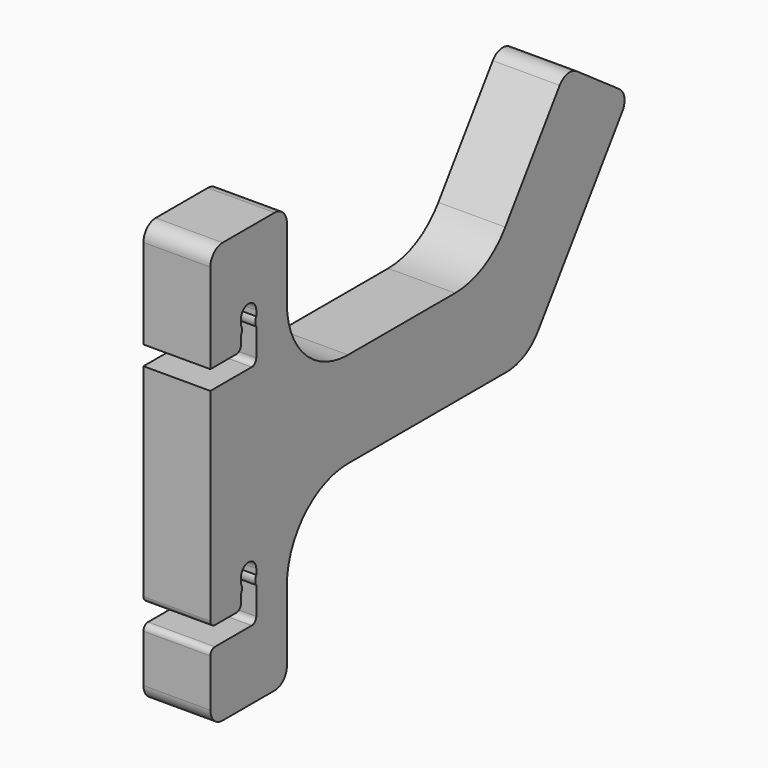
from build123d import *

# Parameters (mm, degrees)
F1_DEPTH = 4.445
F2_R     = 2.032
F4_DEPTH = 8.891
F5_R     = 0.762
F7_DEPTH = 8.89


# Not quite as in the source:
# - a feature names something its author has since deleted; it is built from what else it names


with BuildPart() as f1:
    # F0 (on Right) → F1 (new body, symmetric)
    with BuildSketch(Plane.YZ):
        with BuildLine():
            Line((12.7, 27.94), (0, 27.94))
            Line((0, 27.94), (0, -27.94))
            Line((0, -27.94), (12.7, -27.94))
            Line((12.7, -27.94), (12.7, -16.51))
            ThreePointArc((12.7, -16.51), (15.6757951031, -9.3257951031), (22.86, -6.35))
            Line((22.86, -6.35), (49.2345620046, -6.35))
            ThreePointArc((49.2345620046, -6.35), (52.1666656987, -5.6325187907), (54.4361774858, -3.6422103708))
            Line((54.4361774858, -3.6422103708), (69.5640047708, 17.9625660125))
            Line((69.5640047708, 17.9625660125), (59.1607738083, 25.2469867541))
            Line((59.1607738083, 25.2469867541), (48.96258477, 10.6824634067))
            ThreePointArc((48.96258477, 10.6824634067), (45.3313659105, 7.4979699349), (40.64, 6.35))
            Line((40.64, 6.35), (22.86, 6.35))
            ThreePointArc((22.86, 6.35), (15.6757951031, 9.3257951031), (12.7, 16.51))
            Line((12.7, 16.51), (12.7, 27.94))
        make_face()
    extrude(amount=F1_DEPTH, both=True)

    # F2
    f2_edges = [f1.edges().sort_by_distance(p)[0] for p in [
        (0, 12.7, 27.94),
        (0, 59.160774, 25.246987),
        (0, 69.564005, 17.962566),
        (0, 12.7, -27.94),
        (0, 0, -27.94),
        (0, 0, 27.94),
    ]]
    fillet(f2_edges, radius=F2_R)

    # F3 (on face) → F4 (cut, through all)
    with BuildSketch(Plane.YZ.offset(4.445)):
        with BuildLine():
            Line((7.62, 11.43), (7.62, 17.78))
            ThreePointArc((7.62, 17.78), (6.35, 19.05), (5.08, 17.78))
            Line((5.08, 17.78), (5.08, 13.97))
            Line((5.08, 13.97), (0, 13.97))
            Line((0, 13.97), (0, 11.43))
            Line((0, 11.43), (7.62, 11.43))
        make_face()
        with BuildLine():
            Line((7.62, -18.796), (7.62, -12.446))
            ThreePointArc((7.62, -12.446), (6.35, -11.176), (5.08, -12.446))
            Line((5.08, -12.446), (5.08, -16.256))
            Line((5.08, -16.256), (0, -16.256))
            Line((0, -16.256), (0, -18.796))
            Line((0, -18.796), (7.62, -18.796))
        make_face()
    extrude(amount=-F4_DEPTH, mode=Mode.SUBTRACT)

    # F5
    f5_edges = [f1.edges().sort_by_distance(p)[0] for p in [
        (0, 7.62, 11.43),
        (0, 0, -16.256),
        (0, 7.62, -18.796),
        (0, 0, -18.796),
        (0, 5.08, -16.256),
        (0, 5.08, 13.97),
    ]]
    fillet(f5_edges, radius=F5_R)

    # F6 (on face) → F7 (join, through all)
    with BuildSketch(Plane.YZ.offset(4.445)):
        with BuildLine():
            Line((5.08, 17.0451861632), (5.08, 15.8510145557))
            ThreePointArc((5.08, 15.8510145557), (5.2483526058, 16.4481003594), (5.08, 17.0451861632))
        make_face()
        with BuildLine():
            Line((5.08, -13.1808138368), (5.08, -14.3749854443))
            ThreePointArc((5.08, -14.3749854443), (5.2483526058, -13.7778996406), (5.08, -13.1808138368))
        make_face()
        with BuildLine():
            Line((7.62, -14.3749854443), (7.62, -13.1808138368))
            ThreePointArc((7.62, -13.1808138368), (7.4516473942, -13.7778996406), (7.62, -14.3749854443))
        make_face()
        with BuildLine():
            Line((7.62, 15.8510145557), (7.62, 17.0451861632))
            ThreePointArc((7.62, 17.0451861632), (7.4516473942, 16.4481003594), (7.62, 15.8510145557))
        make_face()
    extrude(amount=-F7_DEPTH)


solid = f1.part
